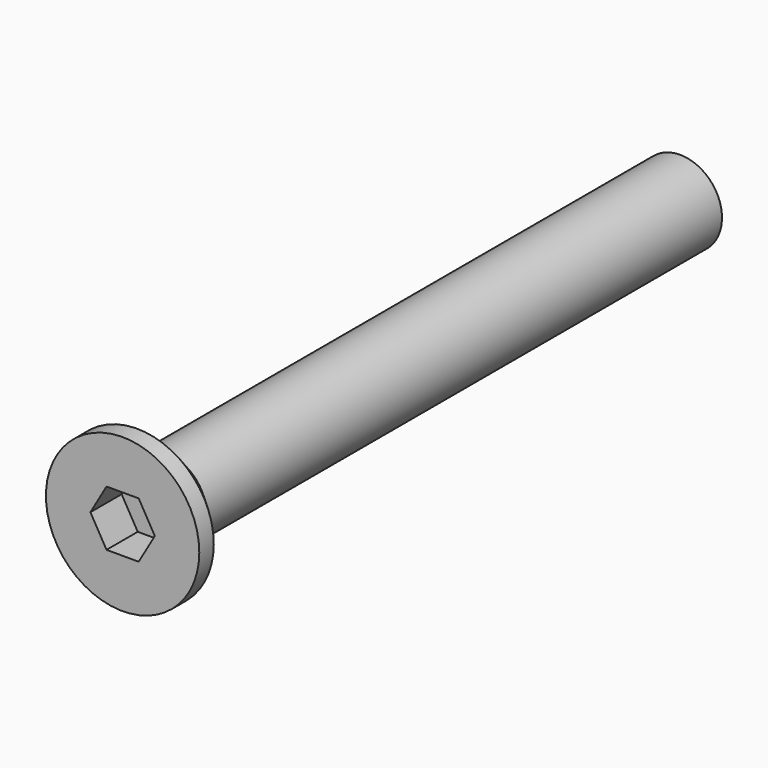
from build123d import *

# Parameters (mm, degrees)
F0_R     = 2.75
F1_DEPTH = 1.9
F2_R     = 1.5
F3_DEPTH = 23.1
F5_START = 0.5
F5_DEPTH = 4.5
F6_SIZE2 = 1.24999
F6_SIZE  = 1.24999


# Not quite as in the source:
# - a fillet or chamfer is up to 0.001 mm smaller than in the source, because OpenCascade refuses the exact size


with BuildPart() as f1:
    # F0 (on Front) → F1 (new body)
    with BuildSketch(Plane.XZ):
        Circle(F0_R)
    extrude(amount=F1_DEPTH)

    # F2 (on face) → F3 (join)
    with BuildSketch(Plane(origin=(0, 0, 0), x_dir=(-1, 0, 0), z_dir=(0, 1, 0))):
        Circle(F2_R)
    extrude(amount=F3_DEPTH)

    # F4 (on Front) → F5 (cut)
    with BuildSketch(Plane.XZ.offset(F5_START)):
        Polygon((1.1547005384, 0), (0.5773502692, 1), (-0.5773502692, 1), (-1.1547005384, 0), (-0.5773502692, -1), (0.5773502692, -1), align=None)
    extrude(amount=F5_DEPTH, mode=Mode.SUBTRACT)

    # F6 (size 1.25 and 1.25 in the source; OpenCascade refuses exactly that, so slightly less here)
    f6_edges = [f1.edges().sort_by_distance(p)[0] for p in [
        (-2.75, 0, 0),
    ]]
    chamfer(f6_edges, length=F6_SIZE, length2=F6_SIZE2)


solid = f1.part
